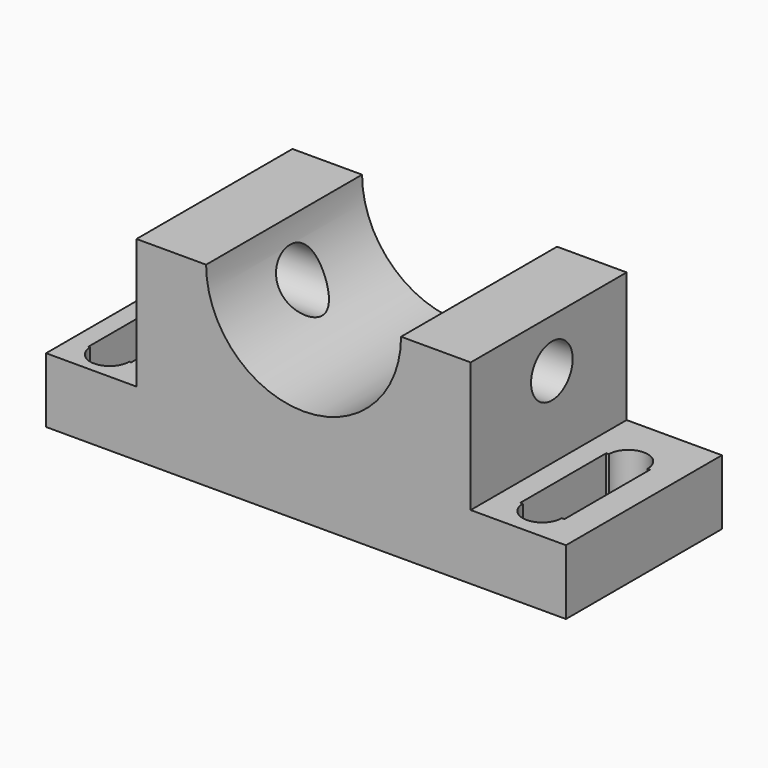
from build123d import *

# Parameters (mm, degrees)
F1_DEPTH = 600
F2_R     = 80
F3_DEPTH = 1321.7481718788
F5_DEPTH = 200.001
F6_DEPTH = 200.001


# Not quite as in the source:
# - a feature names something its author has since deleted; it is built from what else it names


with BuildPart() as f1:
    # F0 (on Front) → F1 (new body)
    with BuildSketch(Plane.XZ):
        with BuildLine():
            Line((506.8030357361, -100), (506.8030357361, 300))
            Line((506.8030357361, 300), (292.5279319286, 300))
            ThreePointArc((292.5279319286, 300), (-7.4720680714, 0), (-307.4720680714, 300))
            Line((-307.4720680714, 300), (-521.7471718788, 300))
            Line((-521.7471718788, 300), (-521.7471718788, -100))
            Line((-521.7471718788, -100), (-800, -100))
            Line((-800, -100), (-800, -300))
            Line((-800, -300), (800, -300))
            Line((800, -300), (800, -100))
            Line((800, -100), (506.8030357361, -100))
        make_face()
    extrude(amount=F1_DEPTH)

    # F2 (on face) → F3 (cut, through all)
    with BuildSketch(Plane(origin=(-521.7471718788, 0, 0), x_dir=(0, -1, 0), z_dir=(-1, 0, 0))):
        with Locations((287.7135872841, 150)):
            Circle(F2_R)
    extrude(amount=-F3_DEPTH, mode=Mode.SUBTRACT)

    # F4 (on face) → F5 (cut, through all)
    with BuildSketch(Plane.XY.offset(-100)):
        with BuildLine():
            Line((-610.4801893234, -509.8910629749), (-610.4801893234, -165.6369864941))
            Line((-610.4801893234, -165.6369864941), (-616.1602163315, -165.6369864941))
            ThreePointArc((-616.1602163315, -165.6369864941), (-676.1602163315, -105.6369864941), (-736.1602163315, -165.6369864941))
            Line((-736.1602163315, -165.6369864941), (-741.8402433395, -165.6369864941))
            Line((-741.8402433395, -165.6369864941), (-741.8402433395, -509.8910629749))
            Line((-741.8402433395, -509.8910629749), (-736.1602163315, -509.8910629749))
            ThreePointArc((-736.1602163315, -509.8910629749), (-676.1602163315, -569.8910629749), (-616.1602163315, -509.8910629749))
            Line((-616.1602163315, -509.8910629749), (-610.4801893234, -509.8910629749))
        make_face()
        with BuildLine():
            Line((704.2353129387, -496.3020980358), (712.1801376343, -496.3020980358))
            Line((712.1801376343, -496.3020980358), (712.1801376343, -165.6369864941))
            Line((712.1801376343, -165.6369864941), (704.2353129387, -165.6369864941))
            ThreePointArc((704.2353129387, -165.6369864941), (644.2353129387, -105.6369864941), (584.2353129387, -165.6369864941))
            Line((584.2353129387, -165.6369864941), (576.2904882431, -165.6369864941))
            Line((576.2904882431, -165.6369864941), (576.2904882431, -496.3020980358))
            Line((576.2904882431, -496.3020980358), (584.2353129387, -496.3020980358))
            ThreePointArc((584.2353129387, -496.3020980358), (644.2353129387, -556.3020980358), (704.2353129387, -496.3020980358))
        make_face()
    extrude(amount=-F5_DEPTH, mode=Mode.SUBTRACT)

    # F4 (on face) → F6 (cut, through all)
    with BuildSketch(Plane.XY.offset(-100)):
        with BuildLine():
            Line((-610.4801893234, -509.8910629749), (-610.4801893234, -165.6369864941))
            Line((-610.4801893234, -165.6369864941), (-616.1602163315, -165.6369864941))
            ThreePointArc((-616.1602163315, -165.6369864941), (-676.1602163315, -105.6369864941), (-736.1602163315, -165.6369864941))
            Line((-736.1602163315, -165.6369864941), (-741.8402433395, -165.6369864941))
            Line((-741.8402433395, -165.6369864941), (-741.8402433395, -509.8910629749))
            Line((-741.8402433395, -509.8910629749), (-736.1602163315, -509.8910629749))
            ThreePointArc((-736.1602163315, -509.8910629749), (-676.1602163315, -569.8910629749), (-616.1602163315, -509.8910629749))
            Line((-616.1602163315, -509.8910629749), (-610.4801893234, -509.8910629749))
        make_face()
        with BuildLine():
            Line((704.2353129387, -496.3020980358), (712.1801376343, -496.3020980358))
            Line((712.1801376343, -496.3020980358), (712.1801376343, -165.6369864941))
            Line((712.1801376343, -165.6369864941), (704.2353129387, -165.6369864941))
            ThreePointArc((704.2353129387, -165.6369864941), (644.2353129387, -105.6369864941), (584.2353129387, -165.6369864941))
            Line((584.2353129387, -165.6369864941), (576.2904882431, -165.6369864941))
            Line((576.2904882431, -165.6369864941), (576.2904882431, -496.3020980358))
            Line((576.2904882431, -496.3020980358), (584.2353129387, -496.3020980358))
            ThreePointArc((584.2353129387, -496.3020980358), (644.2353129387, -556.3020980358), (704.2353129387, -496.3020980358))
        make_face()
    extrude(amount=-F6_DEPTH, mode=Mode.SUBTRACT)


solid = f1.part
